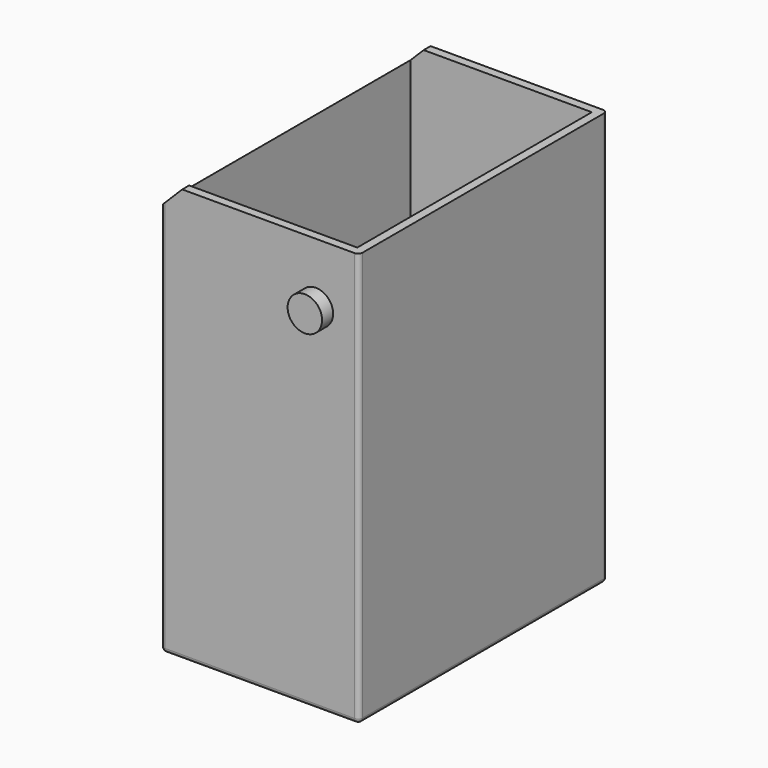
from build123d import *

# Parameters (mm, degrees)
F0_W        = 46
F0_H        = 72
F1_DEPTH    = 96
F2_W        = 42
F2_H        = 68
F3_DEPTH    = 92
F4_R        = 4
F5_DEPTH    = 3.2
F6_R        = 4
F7_DEPTH    = 3.2
F8_T1_DEPTH = 97.7168298797
F9_R        = 1
F10_R       = 27.7209608442
F11_DEPTH   = 2


# Not quite as in the source:
# - a fillet or chamfer that OpenCascade refuses, or shapes differently, is made with other operations: its cross-section is extruded or revolved along the edge and cut away or added


with BuildPart() as f1:
    # F0 (on Top) → F1 (new body)
    with BuildSketch(Plane.XY):
        Rectangle(F0_W, F0_H)
    extrude(amount=F1_DEPTH)

    # F2 (on face) → F3 (cut)
    with BuildSketch(Plane.XY.offset(96)):
        Rectangle(F2_W, F2_H)
    extrude(amount=-F3_DEPTH, mode=Mode.SUBTRACT)

    # F4 (on face) → F5 (join)
    with BuildSketch(Plane.XZ.offset(36)):
        with Locations((13, 82)):
            Circle(F4_R)
    extrude(amount=F5_DEPTH)

    # F6 (on face) → F7 (join)
    with BuildSketch(Plane(origin=(0, 36, 0), x_dir=(-1, 0, 0), z_dir=(0, 1, 0))):
        with Locations((-13, 82)):
            Circle(F6_R)
    extrude(amount=F7_DEPTH)

    # F8: chamfer of 5 on 1 edges, made by hand

    # F8_s2 → F8_t1 (cut)
    with BuildSketch(Plane.XZ.offset(-48.8584149398)):
        Polygon((-18, 96), (-23, 91), (-23, 96), align=None)
    extrude(amount=F8_T1_DEPTH, mode=Mode.SUBTRACT)

    # F9
    f9_edges = [f1.edges().sort_by_distance(p)[0] for p in [
        (-23, -36, 45.5),
        (23, -36, 48),
        (23, 36, 48),
        (-23, 36, 45.5),
        (23, 0, 0),
        (-23, 0, 0),
        (0, 36, 0),
        (0, -36, 0),
    ]]
    fillet(f9_edges, radius=F9_R)

    # F10 (on face) → F11 (join)
    with BuildSketch(Plane(origin=(-23, 0, 0), x_dir=(0, -1, 0), z_dir=(-1, 0, 0))):
        with Locations((0, 40.8182404935)):
            Circle(F10_R)
        with BuildLine():
            add(Edge.make_bspline(
                [(-17.8310812866, 24.7516158604), (-18.0416931886, 24.731624497), (-18.6386807496, 24.6684959969), (-19.2717295968, 24.3841029538), (-19.5649090195, 21.6870798509), (-16.5966593688, 21.0684697904), (-15.2211504824, 21.4407750456), (-14.5426337104, 21.7238514822)],
                knots=[0.4132110552, 0.4132110552, 0.4132110552, 0.4132110552, 0.4283251344, 0.4603190645, 0.510541782, 0.5666924956, 0.615415561, 0.615415561, 0.615415561, 0.615415561], degree=3))
            ThreePointArc((-17.8310812866, 24.7516158604), (-8.6054277875, 63.2242776163), (24.0017475812, 40.8182404935))
            ThreePointArc((24.0017475812, 40.8182404935), (22.6894322226, 32.9904980114), (18.8959899976, 26.0187320907))
            add(Edge.make_bspline(
                [(13.5544067846, 21.0101122713), (15.1773683066, 20.8286148298), (18.6415516168, 20.5611168513), (20.2513827461, 23.1969599021), (20.017563928, 26.727985113), (19.3356446095, 26.1886613097), (18.9151411243, 26.0259448267), (18.8959899976, 26.0187320907)],
                knots=[0.4868760993, 0.4868760993, 0.4868760993, 0.4868760993, 0.6035189288, 0.7106541171, 0.8124300784, 0.8685997483, 0.87123087, 0.87123087, 0.87123087, 0.87123087], degree=3))
            ThreePointArc((13.5544067846, 21.0101122713), (-0.6095113038, 16.8242332642), (-14.5426337104, 21.7238514822))
        make_face(mode=Mode.SUBTRACT)
        with BuildLine():
            add(Edge.make_bspline(
                [(-13.1672387943, 47.9557514191), (-13.6789435568, 47.7302779724), (-13.8554780387, 46.5012200329), (-11.906507855, 43.7928351191), (-10.8613262187, 42.8100774548), (-6.4416701192, 46.0388131445), (-5.8697363247, 48.1862573802), (-6.5496625571, 49.5720681387), (-8.0107671732, 47.5720952119), (-12.18493142, 48.3885873933), (-13.1672387943, 47.9557514191)],
                knots=[0, 0, 0, 0, 0.0951179589, 0.2427295185, 0.3289680533, 0.5102542132, 0.6320447089, 0.7083203168, 0.817404333, 1, 1, 1, 1], degree=3))
        make_face()
        with BuildLine():
            add(Edge.make_bspline(
                [(-1.5056377742, 51.0721281171), (-1.2655745051, 51.376089636), (-0.785072868, 51.9844876136), (0.4890633383, 51.9466317035), (1.1904519521, 51.3741917059), (1.5605587978, 51.0721281171)],
                knots=[0, 0, 0, 0, 0.3204609859, 0.6414226921, 1, 1, 1, 1], degree=3))
            Line((-1.5056377742, 51.0721281171), (-1.5056377742, 40.8182404935))
            Line((-1.5056377742, 40.8182404935), (-13.8206910342, 40.8182404935))
            add(Edge.make_bspline(
                [(-13.8206910342, 40.8182404935), (-14.3163583008, 40.7406958322), (-15.3248298347, 40.5829255117), (-16.0298313022, 38.9853309187), (-15.2661185632, 37.3287424191), (-14.2935212413, 37.5798078265), (-13.8206910342, 37.7018637955)],
                knots=[0, 0, 0, 0, 0.2499158182, 0.5084721255, 0.7610427034, 1, 1, 1, 1], degree=3))
            Line((-13.8206910342, 37.7018637955), (-5.8284727857, 37.7018637955))
            add(Edge.make_bspline(
                [(-5.8284727857, 37.7018637955), (-5.6616792118, 37.7493233921), (-5.1463725609, 37.8959492194), (-5.9050859697, 35.7190459632), (-6.7314491211, 33.7727840823), (-8.8298986523, 30.6803066265), (-10.7443809665, 28.4421062956), (-13.4166866054, 26.493634755), (-15.5645127805, 24.9310548857), (-17.2805677978, 24.8038708143), (-17.8310812866, 24.7516158604)],
                knots=[0, 0, 0, 0, 0.0221816863, 0.0685300411, 0.1230509283, 0.1896466414, 0.2504984271, 0.3136356503, 0.3737047196, 0.4132110552, 0.4132110552, 0.4132110552, 0.4132110552], degree=3))
            ThreePointArc((-17.8310812866, 24.7516158604), (-16.2574965773, 23.1610127385), (-14.5426337104, 21.7238514822))
            add(Edge.make_bspline(
                [(-14.5426337104, 21.7238514822), (-14.4700608663, 21.7541287914), (-13.4868489797, 22.1787471182), (-11.2173445731, 23.4933801542), (-7.8402676501, 26.6128816263), (-5.3447073755, 29.9791410107), (-2.6936822721, 35.9836558885), (-2.3564969432, 37.7686367648), (-1.6866975363, 38.0047224883), (-1.4051069738, 38.1039753556)],
                knots=[0.615415561, 0.615415561, 0.615415561, 0.615415561, 0.620626886, 0.6855816442, 0.7596479515, 0.8338925842, 0.9230870978, 0.9676650246, 1, 1, 1, 1], degree=3))
            Line((-1.4051069738, 38.1039753556), (1.3092315057, 38.1039753556))
            Line((1.3092315057, 38.1039753556), (1.3092315057, 23.5273707658))
            add(Edge.make_bspline(
                [(1.3092315057, 23.5273707658), (1.3901833114, 23.1062891887), (1.5582802327, 22.2319107086), (3.1836032161, 22.2640424108), (4.3821273184, 21.9811997778), (8.5768144522, 21.4369863905), (10.9865964285, 21.3213558963), (13.0868251542, 21.0624024017), (13.5544067846, 21.0101122713)],
                knots=[0, 0, 0, 0, 0.0661108801, 0.1372796485, 0.2082189036, 0.3308717094, 0.453270839, 0.4868760993, 0.4868760993, 0.4868760993, 0.4868760993], degree=3))
            ThreePointArc((13.5544067846, 21.0101122713), (16.4173271562, 23.3095210658), (18.8959899976, 26.0187320907))
            add(Edge.make_bspline(
                [(18.8959899976, 26.0187320907), (17.958719042, 25.6657352116), (16.2187585332, 25.4761750532), (14.4787980244, 25.2866148949)],
                knots=[0.87123087, 0.87123087, 0.87123087, 0.87123087, 1, 1, 1, 1], degree=3))
            Line((14.4787980244, 25.2866148949), (4.274897743, 25.2866148949))
            Line((4.274897743, 25.2866148949), (4.274897743, 38.1039753556))
            Line((4.274897743, 38.1039753556), (14.4787980244, 38.1039753556))
            add(Edge.make_bspline(
                [(14.4787980244, 40.8182404935), (15.0214152926, 40.622477907), (15.9634432149, 40.2826180585), (15.9221942597, 39.1563781008), (15.0189015911, 38.4977733041), (14.4787980244, 38.1039753556)],
                knots=[0, 0, 0, 0, 0.3532671261, 0.6133006012, 1, 1, 1, 1], degree=3))
            Line((14.4787980244, 40.8182404935), (1.5605587978, 40.8182404935))
            Line((1.5605587978, 40.8182404935), (1.5605587978, 51.0721281171))
        make_face()
        with BuildLine():
            add(Edge.make_bspline(
                [(7.2405622341, 48.9107705653), (8.1951903629, 48.5928249221), (11.5971201687, 47.54062061), (13.8463110022, 46.6584207463), (12.1718507315, 44.887582687), (9.6429349022, 43.7513572457), (7.7599373396, 45.9568749284), (7.1288066509, 47.6332666706), (5.7942155786, 48.3483342452), (6.4651933332, 49.1853042153), (6.8443509441, 49.0427315348), (7.2405622341, 48.9107705653)],
                knots=[0, 0, 0, 0, 0.1778305446, 0.288661815, 0.3983430252, 0.5286875411, 0.6581067636, 0.7710159609, 0.8598240036, 0.9261927579, 1, 1, 1, 1], degree=3))
        make_face()
        with BuildLine():
            ThreePointArc((-14.5426337104, 21.7238514822), (-16.2574965773, 23.1610127385), (-17.8310812866, 24.7516158604))
            add(Edge.make_bspline(
                [(-17.8310812866, 24.7516158604), (-18.0416931886, 24.731624497), (-18.6386807496, 24.6684959969), (-19.2717295968, 24.3841029538), (-19.5649090195, 21.6870798509), (-16.5966593688, 21.0684697904), (-15.2211504824, 21.4407750456), (-14.5426337104, 21.7238514822)],
                knots=[0.4132110552, 0.4132110552, 0.4132110552, 0.4132110552, 0.4283251344, 0.4603190645, 0.510541782, 0.5666924956, 0.615415561, 0.615415561, 0.615415561, 0.615415561], degree=3))
        make_face()
        with BuildLine():
            ThreePointArc((18.8959899976, 26.0187320907), (16.4173271562, 23.3095210658), (13.5544067846, 21.0101122713))
            add(Edge.make_bspline(
                [(13.5544067846, 21.0101122713), (15.1773683066, 20.8286148298), (18.6415516168, 20.5611168513), (20.2513827461, 23.1969599021), (20.017563928, 26.727985113), (19.3356446095, 26.1886613097), (18.9151411243, 26.0259448267), (18.8959899976, 26.0187320907)],
                knots=[0.4868760993, 0.4868760993, 0.4868760993, 0.4868760993, 0.6035189288, 0.7106541171, 0.8124300784, 0.8685997483, 0.87123087, 0.87123087, 0.87123087, 0.87123087], degree=3))
        make_face()
    extrude(amount=F11_DEPTH)


solid = f1.part
